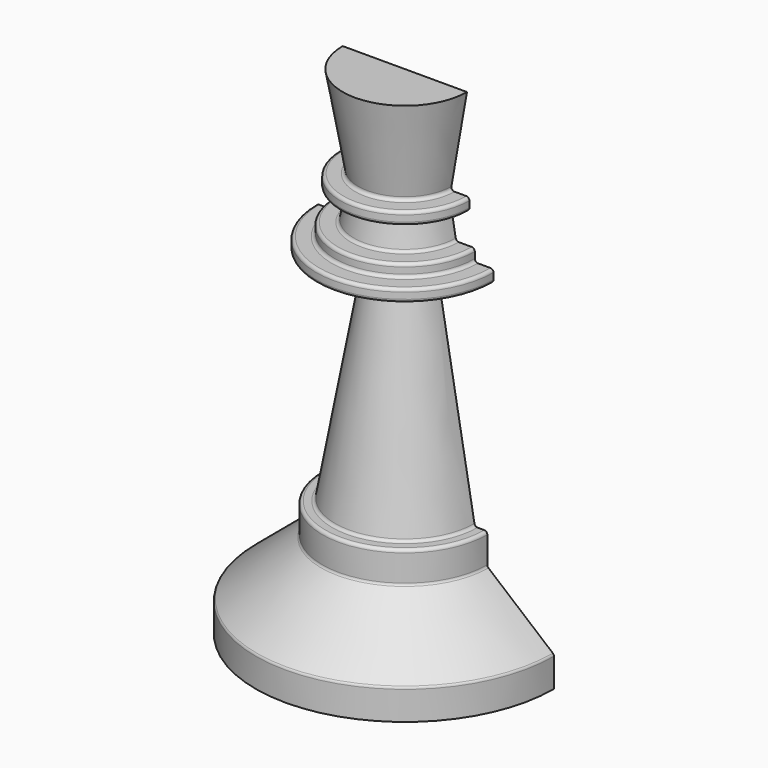
from build123d import *

# Parameters (mm, degrees)
F1_ANGLE = 180


# Not quite as in the source:
# - a feature of the source that left no trace in its solid (it failed there, or was rolled back) is left out


with BuildPart() as f1:
    # F0 (on Front) → F1 (revolve)
    with BuildSketch(Plane.XZ):
        with BuildLine():
            Line((-15.24, 0), (0, 0))
            Line((0, 0), (0, 50.8))
            Line((0, 50.8), (-6.35, 50.8))
            Line((-6.35, 50.8), (-4.7617064118, 41.792339449))
            ThreePointArc((-4.7617064118, 41.792339449), (-4.8311637627, 41.5331210865), (-5.0743828734, 41.4197061526))
            Line((-5.0743828734, 41.4197061526), (-6.2835011077, 41.4197061526))
            ThreePointArc((-6.2835011077, 41.4197061526), (-6.5080075107, 41.3267125556), (-6.6010011077, 41.1022061526))
            Line((-6.6010011077, 41.1022061526), (-6.6010011077, 40.4672061526))
            ThreePointArc((-6.6010011077, 40.4672061526), (-6.5080075107, 40.2426997495), (-6.2835011077, 40.1497061526))
            Line((-6.2835011077, 40.1497061526), (-5.0743828734, 40.1497061526))
            ThreePointArc((-5.0743828734, 40.1497061526), (-4.8311637627, 40.0362912186), (-4.7617064118, 39.7770728561))
            Line((-4.7617064118, 39.7770728561), (-5.2010717431, 37.2853082403))
            ThreePointArc((-5.2010717431, 37.2853082403), (-5.3096631386, 37.0972224261), (-5.5137482047, 37.0229415367))
            Line((-5.5137482047, 37.0229415367), (-6.8348340718, 37.0229415367))
            ThreePointArc((-6.8348340718, 37.0229415367), (-7.0593404748, 36.9299479398), (-7.1523340718, 36.7054415367))
            Line((-7.1523340718, 36.7054415367), (-7.1523340718, 36.0704415367))
            ThreePointArc((-7.1523340718, 36.0704415367), (-7.2453276688, 35.8459351337), (-7.4698340718, 35.7529415367))
            Line((-7.4698340718, 35.7529415367), (-8.7398340718, 35.7529415367))
            ThreePointArc((-8.7398340718, 35.7529415367), (-8.9643404748, 35.6599479398), (-9.0573340718, 35.4354415367))
            Line((-9.0573340718, 35.4354415367), (-9.0573340718, 34.8004415367))
            ThreePointArc((-9.0573340718, 34.8004415367), (-8.9643404748, 34.5759351337), (-8.7398340718, 34.4829415367))
            Line((-8.7398340718, 34.4829415367), (-3.5686493249, 34.4829415367))
            ThreePointArc((-3.5686493249, 34.4829415367), (-3.3254302142, 34.3695266028), (-3.2559728633, 34.1103082403))
            Line((-3.2559728633, 34.1103082403), (-7.113602572, 12.2326030065))
            ThreePointArc((-7.113602572, 12.2326030065), (-7.2221939675, 12.0445171922), (-7.4262790336, 11.9702363029))
            Line((-7.4262790336, 11.9702363029), (-8.1123649007, 11.9702363029))
            ThreePointArc((-8.1123649007, 11.9702363029), (-8.3368713037, 11.8772427059), (-8.4298649007, 11.6527363029))
            Line((-8.4298649007, 11.6527363029), (-8.4298649007, 8.9432889844))
            ThreePointArc((-8.4298649007, 8.9432889844), (-8.4596121783, 8.8091076862), (-8.5432798346, 8.7000698737))
            Line((-8.5432798346, 8.7000698737), (-15.1265850661, 3.176020882))
            ThreePointArc((-15.1265850661, 3.176020882), (-15.2102527224, 3.0669830694), (-15.24, 2.9328017713))
            Line((-15.24, 2.9328017713), (-15.24, 0))
        make_face()
    revolve(axis=Axis((0, 0, 25.4), (0, 0, 1)), revolution_arc=F1_ANGLE)


solid = f1.part
